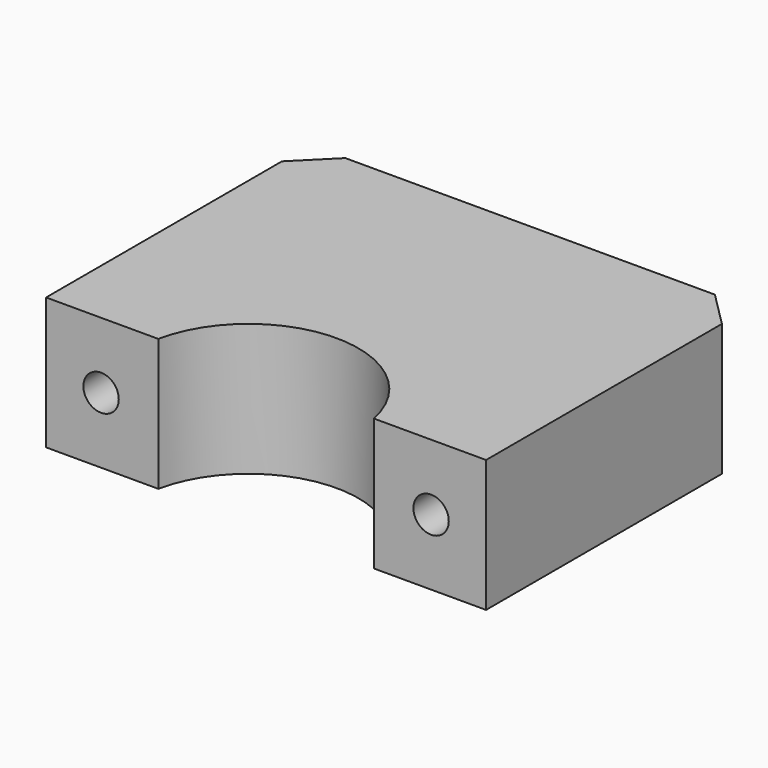
from build123d import *

# Parameters (mm, degrees)
F1_DEPTH = 19.05
F3_D     = 5.1054
F4_SIZE  = 5.08
F6_DEPTH = 25.4
F8_D     = 7.9375
F8_DEPTH = 17.4752
F8_TIP   = 2.3846655818


with BuildPart() as f1:
    # F0 (on Top) → F1 (new body)
    with BuildSketch(Plane.XY):
        with BuildLine():
            Line((0, 50.8), (0, 0))
            Line((0, 0), (15.875, 0))
            ThreePointArc((15.875, 0), (31.75, 15.875), (47.625, 0))
            Line((47.625, 0), (63.5, 0))
            Line((63.5, 0), (63.5, 50.8))
            Line((63.5, 50.8), (0, 50.8))
        make_face()
    extrude(amount=F1_DEPTH)

    # F3 (through all)
    with Locations(Plane(origin=(0, 50.8, 0), x_dir=(-1, 0, 0), z_dir=(0, 1, 0))):
        with Locations((-55.5625, 9.525), (-7.9375, 9.525)):
            Hole(F3_D / 2)

    # F4
    f4_edges = [f1.edges().sort_by_distance(p)[0] for p in [
        (63.5, 50.8, 9.525),
        (0, 50.8, 9.525),
    ]]
    chamfer(f4_edges, length=F4_SIZE)

    # F5 (on face) → F6 (cut)
    with BuildSketch(Plane.XY.offset(19.05)):
        with BuildLine():
            Line((0, 3.175), (0, 0))
            Line((0, 0), (15.875, 0))
            ThreePointArc((15.875, 0), (15.955388571, 1.5955797718), (16.1957401333, 3.175))
            Line((16.1957401333, 3.175), (0, 3.175))
        make_face()
        with BuildLine():
            ThreePointArc((47.3042598667, 3.175), (47.544611429, 1.5955797718), (47.625, 0))
            Line((47.625, 0), (63.5, 0))
            Line((63.5, 0), (63.5, 3.175))
            Line((63.5, 3.175), (47.3042598667, 3.175))
        make_face()
    extrude(amount=-F6_DEPTH, mode=Mode.SUBTRACT)

    # F8
    with Locations(Plane(origin=(0, 50.8, 0), x_dir=(-1, 0, 0), z_dir=(0, 1, 0))):
        with Locations((-31.75, 9.525)):
            Hole(F8_D / 2, depth=F8_DEPTH)
            with Locations((0, 0, -(F8_DEPTH + F8_TIP / 2))):  # 118° drill point
                Cone(0, F8_D / 2, F8_TIP, mode=Mode.SUBTRACT)


solid = f1.part
